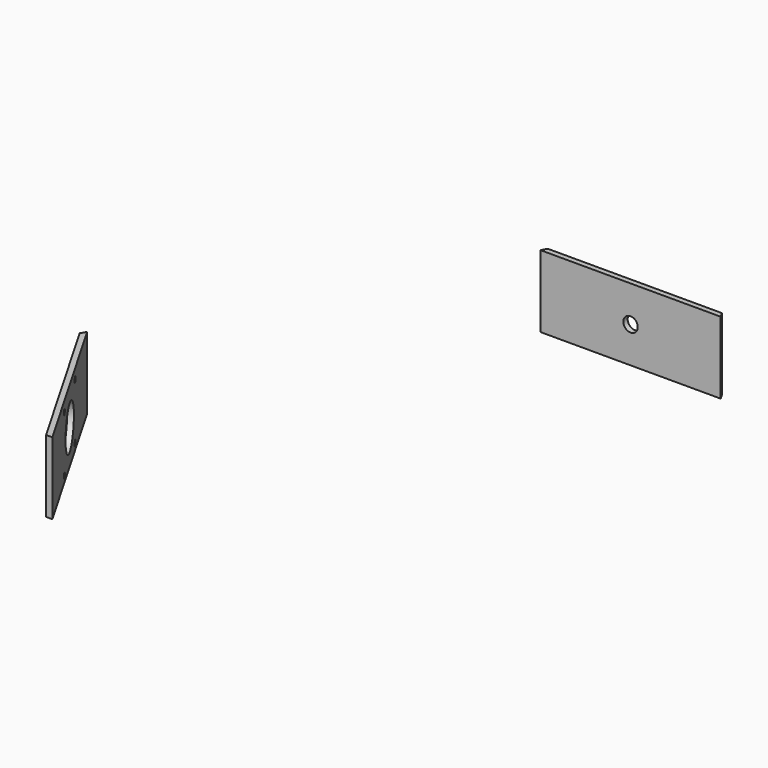
from build123d import *

# Parameters (mm, degrees)
F2_DEPTH = 40
F3_R     = 12
F3_R_2   = 1.5
F4_DEPTH = 25
F5_R     = 4
F6_DEPTH = 25


with BuildPart() as f2:
    # F1 (on face) → F2 (new body)
    with BuildSketch(Plane.XY):
        Polygon((-155.3589838486, -31.9615242271), (-157.0910346562, -34.9615242271), (-108.8230854638, -118.5640646055), (-105.3589838486, -118.5640646055), align=None)
    extrude(amount=F2_DEPTH)

    # F3 (on face) → F4 (cut)
    with BuildSketch(Plane(origin=(-130.3589838486, -75.2627944163, 0), x_dir=(-0.5, 0.8660254038, 0), z_dir=(0.8660254038, 0.5, 0))):
        with Locations((0, 19)):
            Circle(F3_R)
        with Locations((-15.5, 34.5)):
            Circle(F3_R_2)
        with Locations((15.5, 34.5)):
            Circle(F3_R_2)
        with Locations((15.5, 3.5)):
            Circle(F3_R_2)
        with Locations((-15.5, 3.5)):
            Circle(F3_R_2)
    extrude(amount=-F4_DEPTH, mode=Mode.SUBTRACT)


with BuildPart() as f2b:
    # F1 (on face) → F2, piece 2 (new body)
    with BuildSketch(Plane.XY):
        Polygon((-48.2679491924, 153.5255888326), (-50, 150.5255888326), (50, 150.5255888326), (48.2679491924, 153.5255888326), align=None)
    extrude(amount=F2_DEPTH)

    # F5 (on face) → F6 (cut)
    with BuildSketch(Plane.XZ.offset(-150.5255888326)):
        with Locations((0, 20)):
            Circle(F5_R)
    extrude(amount=-F6_DEPTH, mode=Mode.SUBTRACT)


solid = Compound([f2.part, f2b.part])
